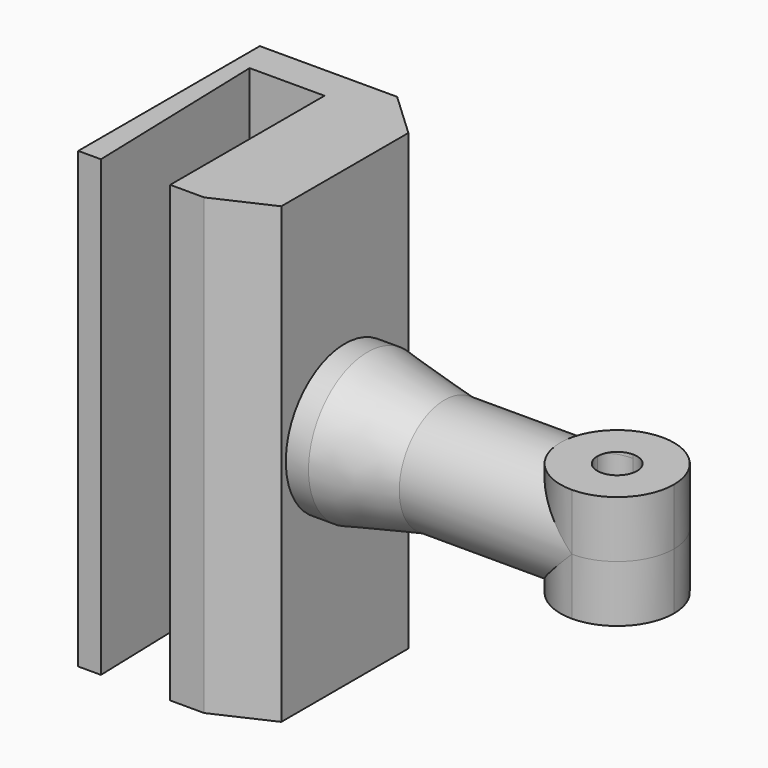
from build123d import *
from build123d import SkipClean  # not in build123d's __all__

# Parameters (mm, degrees)
F1_DEPTH = 20
F0_W     = 2
F0_H     = 6.5
F5_DEPTH = 5
F6_DEPTH = 5


with BuildPart() as f1:
    # F0 (on Top) → F1 (new body, symmetric)
    with BuildSketch(Plane.XY):
        Polygon((-33.9359952807, -3.1263027601), (-33.9359952807, -23.1263027601), (-31.9359952807, -23.1263027601), (-32.4359952807, -6.1263027601), (-25.8359952807, -6.1263027601), (-25.8359952807, -23.1263027601), (-22.8359952807, -23.1263027601), (-17.8684814229, -20.8465269788), (-17.8684814229, -20.3465269788), (-17.8684814229, -13.8465269788), (-17.8684814229, -7.3465269788), (-17.8684814229, -6.8465269788), (-21.8359952807, -3.1263027601), align=None)
    extrude(amount=F1_DEPTH, both=True)

    # F0 (on Top) → F2 (revolve)
    with BuildSketch(Plane.XY):
        with Locations((-16.8684814229, -10.5965269788)):
            Rectangle(F0_W, F0_H)
    revolve(axis=Axis((-16.8684814229, -13.8465269788, 0), (1, 0, 0)))

    # F0 (on Top) → F3 (revolve)
    with BuildSketch(Plane.XY):
        Polygon((-9.0739962115, -8.8465269788), (-15.8684814229, -7.3465269788), (-15.8684814229, -13.8465269788), (-9.0739962115, -13.8465269788), align=None)
    revolve(axis=Axis((-4.8684814229, -13.8465269788, 0), (1, 0, 0)))

    # F0 (on Top) → F4 (revolve)
    with BuildSketch(Plane.XY):
        with BuildLine():
            Line((6.1315185771, -8.8465269788), (-9.0739962115, -8.8465269788))
            Line((-9.0739962115, -8.8465269788), (-9.0739962115, -13.8465269788))
            Line((-9.0739962115, -13.8465269788), (1.1315185771, -13.8465269788))
            ThreePointArc((1.1315185771, -13.8465269788), (2.5959846712, -10.3109930728), (6.1315185771, -8.8465269788))
        make_face()
        with BuildLine():
            Line((6.1315185771, -12.0965269788), (6.1315185771, -8.8465269788))
            ThreePointArc((6.1315185771, -8.8465269788), (2.5959846712, -10.3109930728), (1.1315185771, -13.8465269788))
            Line((1.1315185771, -13.8465269788), (4.3815185771, -13.8465269788))
            ThreePointArc((4.3815185771, -13.8465269788), (4.89408171, -12.6090901117), (6.1315185771, -12.0965269788))
        make_face()
        with BuildLine():
            Line((6.1315185771, -13.8465269788), (6.1315185771, -12.0965269788))
            ThreePointArc((6.1315185771, -12.0965269788), (4.89408171, -12.6090901117), (4.3815185771, -13.8465269788))
            Line((4.3815185771, -13.8465269788), (6.1315185771, -13.8465269788))
        make_face()
    revolve(axis=Axis((-4.8684814229, -13.8465269788, 0), (1, 0, 0)))

    # F0 (on Top) → F5 (cut, symmetric)
    with BuildSketch(Plane.XY):
        with BuildLine():
            Line((6.1315185771, -13.8465269788), (4.3815185771, -13.8465269788))
            ThreePointArc((4.3815185771, -13.8465269788), (4.89408171, -15.0839638459), (6.1315185771, -15.5965269788))
            Line((6.1315185771, -15.5965269788), (6.1315185771, -13.8465269788))
        make_face()
        with BuildLine():
            ThreePointArc((7.8815185771, -13.8465269788), (7.3689554442, -12.6090901117), (6.1315185771, -12.0965269788))
            Line((6.1315185771, -12.0965269788), (6.1315185771, -13.8465269788))
            Line((6.1315185771, -13.8465269788), (6.1315185771, -15.5965269788))
            ThreePointArc((6.1315185771, -15.5965269788), (7.3689554442, -15.0839638459), (7.8815185771, -13.8465269788))
        make_face()
        with BuildLine():
            Line((6.1315185771, -13.8465269788), (6.1315185771, -12.0965269788))
            ThreePointArc((6.1315185771, -12.0965269788), (4.89408171, -12.6090901117), (4.3815185771, -13.8465269788))
            Line((4.3815185771, -13.8465269788), (6.1315185771, -13.8465269788))
        make_face()
    extrude(amount=F5_DEPTH, both=True, mode=Mode.SUBTRACT)

    # F0 (on Top) → F6 (join, symmetric)
    with BuildSketch(Plane.XY):
        with BuildLine():
            Line((6.1315185771, -12.0965269788), (6.1315185771, -8.8465269788))
            ThreePointArc((6.1315185771, -8.8465269788), (2.5959846712, -10.3109930728), (1.1315185771, -13.8465269788))
            Line((1.1315185771, -13.8465269788), (4.3815185771, -13.8465269788))
            ThreePointArc((4.3815185771, -13.8465269788), (4.89408171, -12.6090901117), (6.1315185771, -12.0965269788))
        make_face()
        with BuildLine():
            Line((4.3815185771, -13.8465269788), (1.1315185771, -13.8465269788))
            ThreePointArc((1.1315185771, -13.8465269788), (2.5959846712, -17.3820608847), (6.1315185771, -18.8465269788))
            Line((6.1315185771, -18.8465269788), (6.1315185771, -15.5965269788))
            ThreePointArc((6.1315185771, -15.5965269788), (4.89408171, -15.0839638459), (4.3815185771, -13.8465269788))
        make_face()
        with BuildLine():
            ThreePointArc((11.1315185771, -13.8465269788), (9.667052483, -10.3109930728), (6.1315185771, -8.8465269788))
            Line((6.1315185771, -8.8465269788), (6.1315185771, -12.0965269788))
            ThreePointArc((6.1315185771, -12.0965269788), (7.3689554442, -12.6090901117), (7.8815185771, -13.8465269788))
            ThreePointArc((7.8815185771, -13.8465269788), (7.3689554442, -15.0839638459), (6.1315185771, -15.5965269788))
            Line((6.1315185771, -15.5965269788), (6.1315185771, -18.8465269788))
            ThreePointArc((6.1315185771, -18.8465269788), (9.667052483, -17.3820608847), (11.1315185771, -13.8465269788))
        make_face()
    with SkipClean():  # cleaning this boolean's faces spoils the solid; the shape is the same uncleaned
        extrude(amount=F6_DEPTH, both=True)


solid = f1.part
